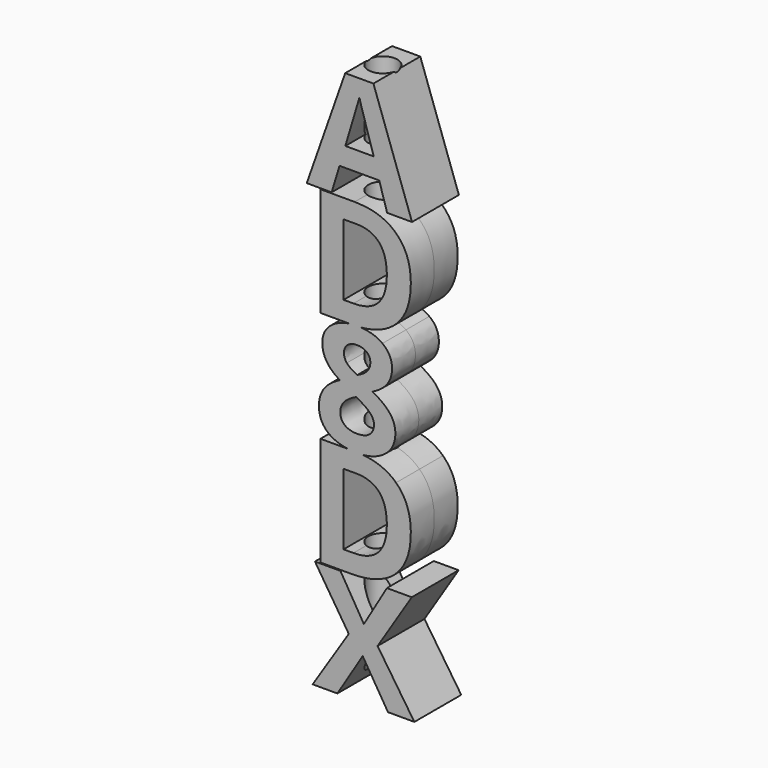
from build123d import *

# Parameters (mm, degrees)
F0_TEXT_SIZE = 41.6666666667
F1_DEPTH     = 8
F3_D         = 7.9375


# Not quite as in the source:
# - a length typed as a fraction of an inch, garbled in the dataset ("3 / 203.2 mm" for 3/8 in), is restored
# - Text() gives the source's letters only with a copy of the font that has no kerning and outlines rounded to 1/6400 em; it was checked with that copy


with BuildPart() as f1:
    # F0 (on Front) → F1 (new body, symmetric)
    with BuildSketch(Plane.XZ):
        with Locations((-14.3850711826, 0)):
            Text('A', F0_TEXT_SIZE, font='Open Sans', font_style=FontStyle.BOLD, text_align=(TextAlign.LEFT, TextAlign.BOTTOM))
        with BuildLine():
            add(Edge.make_bspline(
                [(14.039407984, -14.84375), (14.039407984, -22.1875), (9.8564652757, -26.09375)],
                knots=[0, 0, 0, 1, 1, 1], degree=2))
            add(Edge.make_bspline(
                [(10.0094600674, -4.0983072917), (14.039407984, -7.9427083333), (14.039407984, -14.84375)],
                knots=[0, 0, 0, 1, 1, 1], degree=2))
            add(Edge.make_bspline(
                [(-1.3056440993, -0.25390625), (5.9795121507, -0.25390625), (10.0094600674, -4.0983072917)],
                knots=[0, 0, 0, 1, 1, 1], degree=2))
            Line((-1.3056440993, -0.25390625), (-10.6415815993, -0.25390625))
            Line((-10.6415815993, -0.25390625), (-10.6415815993, -30))
            Line((-10.6415815993, -30), (-2.6772826935, -30))
            add(Edge.make_bspline(
                [(-2.6772826935, -30), (-1.6911922268, -29.8697916667), (-0.5989583333, -29.8697916667)],
                knots=[0.7430825022, 0.7430825022, 0.7430825022, 1, 1, 1], degree=2))
            add(Edge.make_bspline(
                [(-0.5989583333, -29.8697916667), (-0.1390776313, -29.8697916667), (0.3015747326, -29.8922560853)],
                knots=[0, 0, 0, 0.1075154883, 0.1075154883, 0.1075154883], degree=2))
            add(Edge.make_bspline(
                [(9.8564652757, -26.09375), (6.3682241279, -29.351251461), (0.3015747326, -29.8922560853)],
                knots=[0, 0, 0, 0.833920374, 0.833920374, 0.833920374], degree=2))
        make_face()
        with BuildLine():
            add(Edge.make_bspline(
                [(7.4834184007, -15.0065104167), (7.4834184007, -5.4231770833), (-0.980123266, -5.4231770833)],
                knots=[0, 0, 0, 1, 1, 1], degree=2))
            add(Edge.make_bspline(
                [(-1.6311649326, -24.7916666667), (7.4834184007, -24.7916666667), (7.4834184007, -15.0065104167)],
                knots=[0, 0, 0, 1, 1, 1], degree=2))
            Line((-1.6311649326, -24.7916666667), (-4.3329878493, -24.7916666667))
            Line((-4.3329878493, -24.7916666667), (-4.3329878493, -5.4231770833))
            Line((-4.3329878493, -5.4231770833), (-0.980123266, -5.4231770833))
        make_face(mode=Mode.SUBTRACT)
        with BuildLine():
            add(Edge.make_bspline(
                [(0.3015747326, -29.8922560853), (3.9594236235, -30.0787328989), (6.2923177083, -31.8131510417)],
                knots=[0.1075154883, 0.1075154883, 0.1075154883, 1, 1, 1], degree=2))
            add(Edge.make_bspline(
                [(0.3015747326, -29.8922560853), (-0.9066303838, -30), (-2.2171024326, -30)],
                knots=[0.833920374, 0.833920374, 0.833920374, 1, 1, 1], degree=2))
            Line((-2.2171024326, -30), (-2.6772826935, -30))
            add(Edge.make_bspline(
                [(-7.4934895833, -31.8424479167), (-5.5293522402, -30.3766015744), (-2.6772826935, -30)],
                knots=[0, 0, 0, 0.7430825022, 0.7430825022, 0.7430825022], degree=2))
            add(Edge.make_bspline(
                [(-10.13671875, -37.01171875), (-10.13671875, -33.8151041667), (-7.4934895833, -31.8424479167)],
                knots=[0, 0, 0, 1, 1, 1], degree=2))
            add(Edge.make_bspline(
                [(-9.0201822917, -41.0188802083), (-10.13671875, -39.1861979167), (-10.13671875, -37.01171875)],
                knots=[0, 0, 0, 1, 1, 1], degree=2))
            add(Edge.make_bspline(
                [(-5.3580729167, -44.453125), (-7.9036458333, -42.8515625), (-9.0201822917, -41.0188802083)],
                knots=[0, 0, 0, 1, 1, 1], degree=2))
            add(Edge.make_bspline(
                [(-9.7005208333, -47.9361979167), (-8.3463541667, -45.9635416667), (-5.3580729167, -44.453125)],
                knots=[0, 0, 0, 1, 1, 1], degree=2))
            add(Edge.make_bspline(
                [(-11.0546875, -52.4544270833), (-11.0546875, -49.9088541667), (-9.7005208333, -47.9361979167)],
                knots=[0, 0, 0, 1, 1, 1], degree=2))
            add(Edge.make_bspline(
                [(-8.2682291667, -58.3333333333), (-11.0546875, -56.2565104167), (-11.0546875, -52.4544270833)],
                knots=[0, 0, 0, 1, 1, 1], degree=2))
            add(Edge.make_bspline(
                [(-3.119854059, -60.25390625), (-6.2460690261, -59.8405040923), (-8.2682291667, -58.3333333333)],
                knots=[0.2742901925, 0.2742901925, 0.2742901925, 1, 1, 1], degree=2))
            Line((-3.119854059, -60.25390625), (-1.3056440993, -60.25390625))
            add(Edge.make_bspline(
                [(-1.3056440993, -60.25390625), (-0.160818529, -60.25390625), (0.9036211763, -60.3488419565)],
                knots=[0, 0, 0, 0.1571449576, 0.1571449576, 0.1571449576], degree=2))
            add(Edge.make_bspline(
                [(6.9498697917, -58.1803385417), (4.5575863912, -60.0403999824), (0.9036211763, -60.3488419565)],
                knots=[0, 0, 0, 0.8341764593, 0.8341764593, 0.8341764593], degree=2))
            add(Edge.make_bspline(
                [(9.8177083333, -52.2916666667), (9.8177083333, -55.9505208333), (6.9498697917, -58.1803385417)],
                knots=[0, 0, 0, 1, 1, 1], degree=2))
            add(Edge.make_bspline(
                [(8.3626302083, -48.0240885417), (9.8177083333, -49.9674479167), (9.8177083333, -52.2916666667)],
                knots=[0, 0, 0, 1, 1, 1], degree=2))
            add(Edge.make_bspline(
                [(3.57421875, -44.2903645833), (6.9075520833, -46.0807291667), (8.3626302083, -48.0240885417)],
                knots=[0, 0, 0, 1, 1, 1], degree=2))
            add(Edge.make_bspline(
                [(7.6432291667, -41.1100260417), (6.3802083333, -42.890625), (3.57421875, -44.2903645833)],
                knots=[0, 0, 0, 1, 1, 1], degree=2))
            add(Edge.make_bspline(
                [(8.90625, -37.05078125), (8.90625, -39.3294270833), (7.6432291667, -41.1100260417)],
                knots=[0, 0, 0, 1, 1, 1], degree=2))
            add(Edge.make_bspline(
                [(6.2923177083, -31.8131510417), (8.90625, -33.7565104167), (8.90625, -37.05078125)],
                knots=[0, 0, 0, 1, 1, 1], degree=2))
        make_face()
        with BuildLine():
            add(Edge.make_bspline(
                [(-5.234375, -52.0833333333), (-5.234375, -53.8346354167), (-4.013671875, -54.8111979167)],
                knots=[0, 0, 0, 1, 1, 1], degree=2))
            add(Edge.make_bspline(
                [(-0.9049479167, -47.0377604167), (-5.234375, -49.0364583333), (-5.234375, -52.0833333333)],
                knots=[0, 0, 0, 1, 1, 1], degree=2))
            add(Edge.make_bspline(
                [(2.8287760417, -49.5735677083), (1.6796875, -48.3854166667), (-0.9049479167, -47.0377604167)],
                knots=[0, 0, 0, 1, 1, 1], degree=2))
            add(Edge.make_bspline(
                [(3.9778645833, -52.12890625), (3.9778645833, -50.76171875), (2.8287760417, -49.5735677083)],
                knots=[0, 0, 0, 1, 1, 1], degree=2))
            add(Edge.make_bspline(
                [(2.8190104167, -54.7819010417), (3.9778645833, -53.7760416667), (3.9778645833, -52.12890625)],
                knots=[0, 0, 0, 1, 1, 1], degree=2))
            add(Edge.make_bspline(
                [(-0.6770833333, -55.7877604167), (1.66015625, -55.7877604167), (2.8190104167, -54.7819010417)],
                knots=[0, 0, 0, 1, 1, 1], degree=2))
            add(Edge.make_bspline(
                [(-4.013671875, -54.8111979167), (-2.79296875, -55.7877604167), (-0.6770833333, -55.7877604167)],
                knots=[0, 0, 0, 1, 1, 1], degree=2))
        make_face(mode=Mode.SUBTRACT)
        with BuildLine():
            add(Edge.make_bspline(
                [(-0.6380208333, -34.4661458333), (-2.24609375, -34.4661458333), (-3.232421875, -35.2897135417)],
                knots=[0, 0, 0, 1, 1, 1], degree=2))
            add(Edge.make_bspline(
                [(1.9661458333, -35.2799479167), (0.9505208333, -34.4661458333), (-0.6380208333, -34.4661458333)],
                knots=[0, 0, 0, 1, 1, 1], degree=2))
            add(Edge.make_bspline(
                [(2.9817708333, -37.5), (2.9817708333, -36.09375), (1.9661458333, -35.2799479167)],
                knots=[0, 0, 0, 1, 1, 1], degree=2))
            add(Edge.make_bspline(
                [(2.1907552083, -39.7591145833), (2.9817708333, -38.7825520833), (2.9817708333, -37.5)],
                knots=[0, 0, 0, 1, 1, 1], degree=2))
            add(Edge.make_bspline(
                [(-0.5989583333, -41.6666666667), (1.3997395833, -40.7356770833), (2.1907552083, -39.7591145833)],
                knots=[0, 0, 0, 1, 1, 1], degree=2))
            add(Edge.make_bspline(
                [(-3.4342447917, -39.6842447917), (-2.6497395833, -40.6510416667), (-0.5989583333, -41.6666666667)],
                knots=[0, 0, 0, 1, 1, 1], degree=2))
            add(Edge.make_bspline(
                [(-4.21875, -37.5), (-4.21875, -38.7174479167), (-3.4342447917, -39.6842447917)],
                knots=[0, 0, 0, 1, 1, 1], degree=2))
            add(Edge.make_bspline(
                [(-3.232421875, -35.2897135417), (-4.21875, -36.11328125), (-4.21875, -37.5)],
                knots=[0, 0, 0, 1, 1, 1], degree=2))
        make_face(mode=Mode.SUBTRACT)
        with BuildLine():
            add(Edge.make_bspline(
                [(0.3015747326, -29.8922560853), (-0.9066303838, -30), (-2.2171024326, -30)],
                knots=[0.833920374, 0.833920374, 0.833920374, 1, 1, 1], degree=2))
            add(Edge.make_bspline(
                [(-0.5989583333, -29.8697916667), (-0.1390776313, -29.8697916667), (0.3015747326, -29.8922560853)],
                knots=[0, 0, 0, 0.1075154883, 0.1075154883, 0.1075154883], degree=2))
            add(Edge.make_bspline(
                [(-2.6772826935, -30), (-1.6911922268, -29.8697916667), (-0.5989583333, -29.8697916667)],
                knots=[0.7430825022, 0.7430825022, 0.7430825022, 1, 1, 1], degree=2))
            Line((-2.6772826935, -30), (-2.2171024326, -30))
        make_face()
        with BuildLine():
            add(Edge.make_bspline(
                [(0.9036211763, -60.3488419565), (6.6127981454, -60.8580344888), (10.0094600674, -64.0983072917)],
                knots=[0.1571449576, 0.1571449576, 0.1571449576, 1, 1, 1], degree=2))
            add(Edge.make_bspline(
                [(0.9036211763, -60.3488419565), (0.1772599335, -60.41015625), (-0.5989583333, -60.41015625)],
                knots=[0.8341764593, 0.8341764593, 0.8341764593, 1, 1, 1], degree=2))
            add(Edge.make_bspline(
                [(-0.5989583333, -60.41015625), (-1.938265914, -60.41015625), (-3.119854059, -60.25390625)],
                knots=[0, 0, 0, 0.2742901925, 0.2742901925, 0.2742901925], degree=2))
            Line((-3.119854059, -60.25390625), (-10.6415815993, -60.25390625))
            Line((-10.6415815993, -60.25390625), (-10.6415815993, -90))
            Line((-10.6415815993, -90), (-2.2171024326, -90))
            add(Edge.make_bspline(
                [(9.8564652757, -86.09375), (5.6735225674, -90), (-2.2171024326, -90)],
                knots=[0, 0, 0, 1, 1, 1], degree=2))
            add(Edge.make_bspline(
                [(14.039407984, -74.84375), (14.039407984, -82.1875), (9.8564652757, -86.09375)],
                knots=[0, 0, 0, 1, 1, 1], degree=2))
            add(Edge.make_bspline(
                [(10.0094600674, -64.0983072917), (14.039407984, -67.9427083333), (14.039407984, -74.84375)],
                knots=[0, 0, 0, 1, 1, 1], degree=2))
        make_face()
        with BuildLine():
            add(Edge.make_bspline(
                [(7.4834184007, -75.0065104167), (7.4834184007, -65.4231770833), (-0.980123266, -65.4231770833)],
                knots=[0, 0, 0, 1, 1, 1], degree=2))
            add(Edge.make_bspline(
                [(-1.6311649326, -84.7916666667), (7.4834184007, -84.7916666667), (7.4834184007, -75.0065104167)],
                knots=[0, 0, 0, 1, 1, 1], degree=2))
            Line((-1.6311649326, -84.7916666667), (-4.3329878493, -84.7916666667))
            Line((-4.3329878493, -84.7916666667), (-4.3329878493, -65.4231770833))
            Line((-4.3329878493, -65.4231770833), (-0.980123266, -65.4231770833))
        make_face(mode=Mode.SUBTRACT)
        with BuildLine():
            add(Edge.make_bspline(
                [(0.9036211763, -60.3488419565), (0.1772599335, -60.41015625), (-0.5989583333, -60.41015625)],
                knots=[0.8341764593, 0.8341764593, 0.8341764593, 1, 1, 1], degree=2))
            add(Edge.make_bspline(
                [(-1.3056440993, -60.25390625), (-0.160818529, -60.25390625), (0.9036211763, -60.3488419565)],
                knots=[0, 0, 0, 0.1571449576, 0.1571449576, 0.1571449576], degree=2))
            Line((-1.3056440993, -60.25390625), (-3.119854059, -60.25390625))
            add(Edge.make_bspline(
                [(-0.5989583333, -60.41015625), (-1.938265914, -60.41015625), (-3.119854059, -60.25390625)],
                knots=[0, 0, 0, 0.2742901925, 0.2742901925, 0.2742901925], degree=2))
        make_face()
        with Locations((-12.7803412685, -120)):
            Text('X', F0_TEXT_SIZE, font='Open Sans', font_style=FontStyle.BOLD, text_align=(TextAlign.LEFT, TextAlign.BOTTOM))
    extrude(amount=F1_DEPTH, both=True)

    # F3 (through all)
    with Locations(Plane.XY.offset(29.8697916667)):
        with Locations((0, 0)):
            Hole(F3_D / 2)


solid = f1.part
